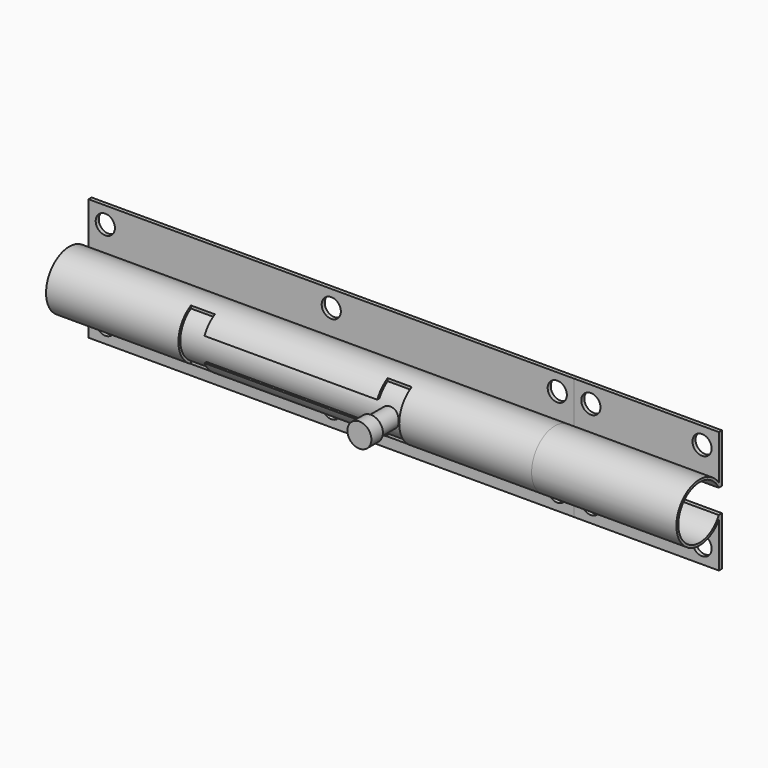
from build123d import *

# Parameters (mm, degrees)
F0_R      = 2
F0_W      = 23
F0_H      = 2.5
F2_DEPTH  = 0.8
F3_DEPTH  = 50.58
F0_W_2    = 30.1626
F0_H_2    = 10.20005
F4_DEPTH  = 0.8
F5_DEPTH  = 30.1626
F6_DEPTH  = 25
F7_DEPTH  = 75
F0_W_3    = 27.58
F0_H_3    = 5
F8_DEPTH  = 2
F10_W     = 5
F10_H     = 5
F11_DEPTH = 5
F12_DEPTH = 25
F13_DEPTH = 50.8
F14_DEPTH = 17.42625
F15_R     = 2
F16_DEPTH = 2.5
F17_R     = 2.5
F17_R_2   = 2.3370450509
F17_R_3   = 2
F18_DEPTH = 3


with BuildPart() as f2:
    # F0 (on Front) → F2 (new body)
    with BuildSketch(Plane.XZ):
        Polygon((50.58, 12.70005), (-50.58, 12.70005), (-50.58, 2.5), (-23, 2.5), (0, 2.5), (23, 2.5), (50.58, 2.5), align=None)
        with Locations((-47.08, 9.20005)):
            Circle(F0_R, mode=Mode.SUBTRACT)
        with BuildLine():
            ThreePointArc((2, 9.20005), (0.9728901826, 7.4526277006), (-1.0534846926, 7.5))
            ThreePointArc((-1.0534846926, 7.5), (-0.9728901826, 10.9474722994), (2, 9.20005))
        make_face(mode=Mode.SUBTRACT)
        with Locations((47.08, 9.20005)):
            Circle(F0_R, mode=Mode.SUBTRACT)
        with Locations((-11.5, -1.25)):
            Rectangle(F0_W, F0_H)
        with Locations((-11.5, 1.25)):
            Rectangle(F0_W, F0_H)
        Polygon((23, -2.5), (23, 2.5), (0, 2.5), (0, 0), (0, -2.5), align=None)
        Polygon((-23, -2.5), (-50.58, -2.5), (-50.58, -12.70005), (50.58, -12.70005), (50.58, -2.5), (23, -2.5), (0, -2.5), align=None)
        with Locations((-47.08, -9.20005)):
            Circle(F0_R, mode=Mode.SUBTRACT)
        with Locations((0, -9.20005)):
            Circle(F0_R, mode=Mode.SUBTRACT)
        with Locations((47.08, -9.20005)):
            Circle(F0_R, mode=Mode.SUBTRACT)
    extrude(amount=-F2_DEPTH)

    # F1 (on Right) → F3 (join, symmetric)
    with BuildSketch(Plane.YZ):
        with BuildLine():
            Line((0.55625, 0), (1.05625, 0))
            ThreePointArc((1.05625, 0), (-5, 6.05625), (-11.05625, 0))
            Line((-11.05625, 0), (-10.55625, 0))
            ThreePointArc((-10.55625, 0), (-5, 5.55625), (0.55625, 0))
        make_face()
        with BuildLine():
            ThreePointArc((-11.05625, 0), (-5, -6.05625), (1.05625, 0))
            Line((1.05625, 0), (0.55625, 0))
            ThreePointArc((0.55625, 0), (-5, -5.55625), (-10.55625, 0))
            Line((-10.55625, 0), (-11.05625, 0))
        make_face()
    extrude(amount=F3_DEPTH, both=True)


with BuildPart() as f4:
    # F0 (on Front) → F4 (new body)
    with BuildSketch(Plane.XZ):
        with Locations((65.6613, 7.600025)):
            Rectangle(F0_W_2, F0_H_2)
        with Locations((54.08, 9.20005)):
            Circle(F0_R, mode=Mode.SUBTRACT)
        with Locations((77.2426, 9.20005)):
            Circle(F0_R, mode=Mode.SUBTRACT)
    extrude(amount=-F4_DEPTH)

    # F5 (add): a face of the model
    f5_faces = [f2.part.faces().sort_by_distance(p)[0] for p in [
        (50.58, 0.2814032225, 8.0586914436),
    ]]


with BuildPart() as f4b:
    # F0 (on Front) → F4, piece 2 (new body)
    with BuildSketch(Plane.XZ):
        with Locations((65.6613, -7.600025)):
            Rectangle(F0_W_2, F0_H_2)
        with Locations((54.08, -9.20005)):
            Circle(F0_R, mode=Mode.SUBTRACT)
        with Locations((77.2426, -9.20005)):
            Circle(F0_R, mode=Mode.SUBTRACT)
    extrude(amount=-F4_DEPTH)


with BuildPart() as f4_1:
    add(f4.part)

    add(f4b.part)  # F5 merges F4b
    extrude(f5_faces, amount=F5_DEPTH)

    # F0 (on Front) → F6 (cut)
    with BuildSketch(Plane.XZ):
        with Locations((54.08, 9.20005)):
            Circle(F0_R)
        with Locations((77.2426, 9.20005)):
            Circle(F0_R)
        with Locations((77.2426, -9.20005)):
            Circle(F0_R)
        with Locations((54.08, -9.20005)):
            Circle(F0_R)
    extrude(amount=-F6_DEPTH, mode=Mode.SUBTRACT)


with BuildPart() as f2_1:
    add(f2.part)

    # F0 (on Front) → F7 (cut, symmetric)
    with BuildSketch(Plane.XZ):
        with Locations((-11.5, -1.25)):
            Rectangle(F0_W, F0_H)
        with Locations((-11.5, 1.25)):
            Rectangle(F0_W, F0_H)
        Polygon((23, -2.5), (23, 2.5), (0, 2.5), (0, 0), (0, -2.5), align=None)
    extrude(amount=F7_DEPTH, both=True, mode=Mode.SUBTRACT)


with BuildPart() as f8_tool:
    # F0 (on Front) → F8 (new body, symmetric)
    with BuildSketch(Plane.XZ):
        Polygon((-23, 2.5), (-50.58, 2.5), (-50.58, -2.5), (-23, -2.5), (-23, 0), align=None)
        with Locations((36.79, 0)):
            Rectangle(F0_W_3, F0_H_3)
        with Locations((65.6613, 0)):
            Rectangle(F0_W_2, F0_H_3)
    extrude(amount=F8_DEPTH, both=True)


with BuildPart() as f2_2:
    add(f2_1.part)

    # F8: cut by f8_tool
    add(f8_tool.part, mode=Mode.SUBTRACT)

    # F10 (on offset) → F11 (cut)
    with BuildSketch(Plane.XZ.offset(12.806)):
        with Locations((-20.5, 5)):
            Rectangle(F10_W, F10_H)
        with Locations((-20.5, -5)):
            Rectangle(F10_W, F10_H)
        with Locations((20.5, 5)):
            Rectangle(F10_W, F10_H)
        with Locations((20.5, -5)):
            Rectangle(F10_W, F10_H)
    extrude(amount=-F11_DEPTH, mode=Mode.SUBTRACT)


with BuildPart() as f4_2:
    add(f4_1.part)

    # F8: cut by f8_tool
    add(f8_tool.part, mode=Mode.SUBTRACT)


with BuildPart() as f12:
    # F1 (on Right) → F12 (new body)
    with BuildSketch(Plane.YZ):
        with BuildLine():
            ThreePointArc((-10.55625, 0), (-5, -5.55625), (0.55625, 0))
            ThreePointArc((0.55625, 0), (-5, 5.55625), (-10.55625, 0))
        make_face()
    extrude(amount=-F12_DEPTH)

    # F1 (on Right) → F13 (join)
    with BuildSketch(Plane.YZ):
        with BuildLine():
            ThreePointArc((-10.55625, 0), (-5, -5.55625), (0.55625, 0))
            ThreePointArc((0.55625, 0), (-5, 5.55625), (-10.55625, 0))
        make_face()
    extrude(amount=F13_DEPTH)

    # F14 (add): a face of the model
    f14_faces = [f12.faces().sort_by_distance(p)[0] for p in [
        (50.8, -5, 0),
    ]]
    extrude(f14_faces, amount=F14_DEPTH)

    # F15 (on offset) → F16 (join, symmetric)
    with BuildSketch(Plane.XZ.offset(12.806)):
        with Locations((20.5, 0)):
            Circle(F15_R)
    extrude(amount=F16_DEPTH, both=True)

    # F17 (on face) → F18 (join)
    with BuildSketch(Plane.XZ.offset(15.306)):
        with Locations((20.5, 0)):
            Circle(F17_R)
        with Locations((20.5, 0)):
            Circle(F17_R_2, mode=Mode.SUBTRACT)
        with Locations((20.5, 0)):
            Circle(F17_R_2)
        with Locations((20.5, 0)):
            Circle(F17_R_3, mode=Mode.SUBTRACT)
        with Locations((20.5, 0)):
            Circle(F17_R_3)
    extrude(amount=F18_DEPTH)


solid = Compound([f2_2.part, f4_2.part, f12.part])
